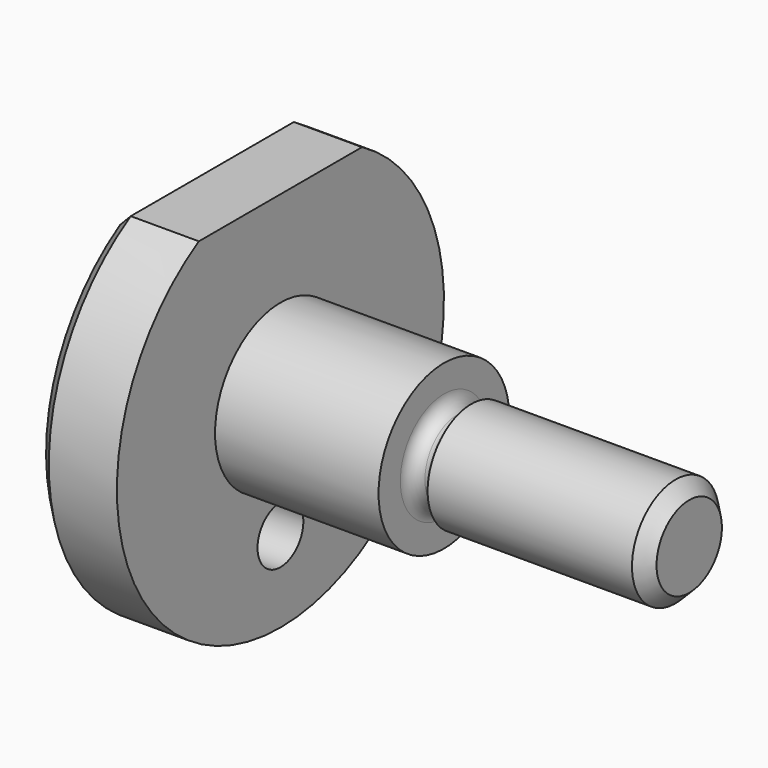
from build123d import *

# Parameters (mm, degrees)
F3_DEPTH = 25
F4_SIZE  = 1
F5_R     = 2.1
F6_DEPTH = 6


with BuildPart() as f1:
    # F0 (on Top) → F1 (revolve)
    with BuildSketch(Plane.XY):
        with BuildLine():
            Line((0, 15), (0, 0))
            Line((0, 0), (36, 0))
            Line((36, 0), (36, 4))
            Line((36, 4), (20, 4))
            ThreePointArc((20, 4), (19.7071067812, 3.2928932188), (19, 3))
            ThreePointArc((19, 3), (18.2928932188, 3.2928932188), (18, 4))
            Line((18, 4), (18, 6))
            Line((18, 6), (6, 6))
            Line((6, 6), (6, 15))
            Line((6, 15), (0, 15))
        make_face()
    revolve(axis=Axis((18, 0, 0), (-1, 0, 0)))

    # F2 (on face) → F3 (cut)
    with BuildSketch(Plane(origin=(0, 0, 0), x_dir=(0, -1, 0), z_dir=(-1, 0, 0))):
        with BuildLine():
            Line((23.4234053642, 26.5963438079), (-25.4426617175, 26.5963438079))
            Line((-25.4426617175, 26.5963438079), (-25.4426617175, 13))
            Line((-25.4426617175, 13), (-7.4833147735, 13))
            ThreePointArc((-7.4833147735, 13), (0, 15), (7.4833147735, 13))
            Line((7.4833147735, 13), (23.4234053642, 13))
            Line((23.4234053642, 13), (23.4234053642, 26.5963438079))
        make_face()
        with BuildLine():
            ThreePointArc((7.4833147735, 13), (0, 15), (-7.4833147735, 13))
            Line((-7.4833147735, 13), (7.4833147735, 13))
        make_face()
    extrude(amount=-F3_DEPTH, mode=Mode.SUBTRACT)

    # F4
    f4_edges = [f1.edges().sort_by_distance(p)[0] for p in [
        (0, 0, -15),
        (0, 0, 13),
        (36, -4, 0),
    ]]
    chamfer(f4_edges, length=F4_SIZE)

    # F5 (on face) → F6 (cut)
    with BuildSketch(Plane(origin=(0, 0, 0), x_dir=(0, -1, 0), z_dir=(-1, 0, 0))):
        with Locations((0, -9)):
            Circle(F5_R)
    extrude(amount=-F6_DEPTH, mode=Mode.SUBTRACT)


solid = f1.part
